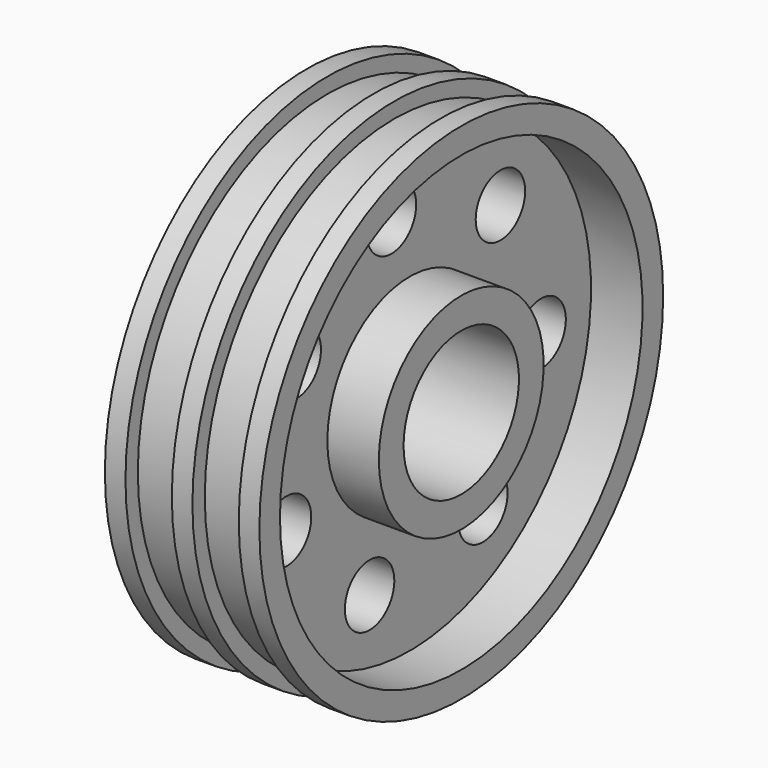
from build123d import *

# Parameters (mm, degrees)
F2_R            = 152.4
F3_DEPTH        = 2230.12
F4_DEPTH        = 508.001
F4_COPIES_COUNT = 7


# Not quite as in the source:
# - a pattern or mirror of a feature is missing from the dataset's text; its kind, count and spacing are read off the source's solid
# - a feature names something its author has since deleted; it is built from what else it names


with BuildPart() as f1:
    # F0 (on Top) → F1 (revolve)
    with BuildSketch(Plane.XY):
        Polygon((381, 812.8), (-381, 812.8), (-381, 660.4), (-127, 660.4), (-127, 50.8), (-381, 50.8), (-381, -76.2), (-279.4, -76.2), (-279.4, 0), (-50.8, 0), (-50.8, -76.2), (0, -76.2), (50.8, -76.2), (50.8, 0), (279.4, 0), (279.4, -76.2), (381, -76.2), (381, 50.8), (127, 50.8), (127, 660.4), (381, 660.4), align=None)
    revolve(axis=Axis((-38.2948741317, 1168.4, 0), (-1, 0, 0)))

    # F2 (on face) → F3 (cut)
    with BuildSketch(Plane(origin=(-127, 0, 0), x_dir=(0, -1, 0), z_dir=(-1, 0, 0))):
        with Locations((-1727.3747412179, 590.0771802742)):
            Circle(F2_R)
    extrude(amount=-F3_DEPTH, mode=Mode.SUBTRACT)

    # F2 (on face) → F4 (cut, through all)
    with BuildSketch(Plane(origin=(-127, 0, 0), x_dir=(0, -1, 0), z_dir=(-1, 0, 0))):
        with Locations((-1727.3747412179, 590.0771802742)):
            Circle(F2_R)
    f4 = extrude(amount=-F4_DEPTH, mode=Mode.SUBTRACT)

    # F4_copies: F4 ×7 about axis
    f4_copies_axis = Axis((0, 1168.4, 0), (1, 0, 0))
    for i in range(1, F4_COPIES_COUNT):
        add(f4.rotate(f4_copies_axis, i * 360 / F4_COPIES_COUNT), mode=Mode.SUBTRACT)


solid = f1.part
